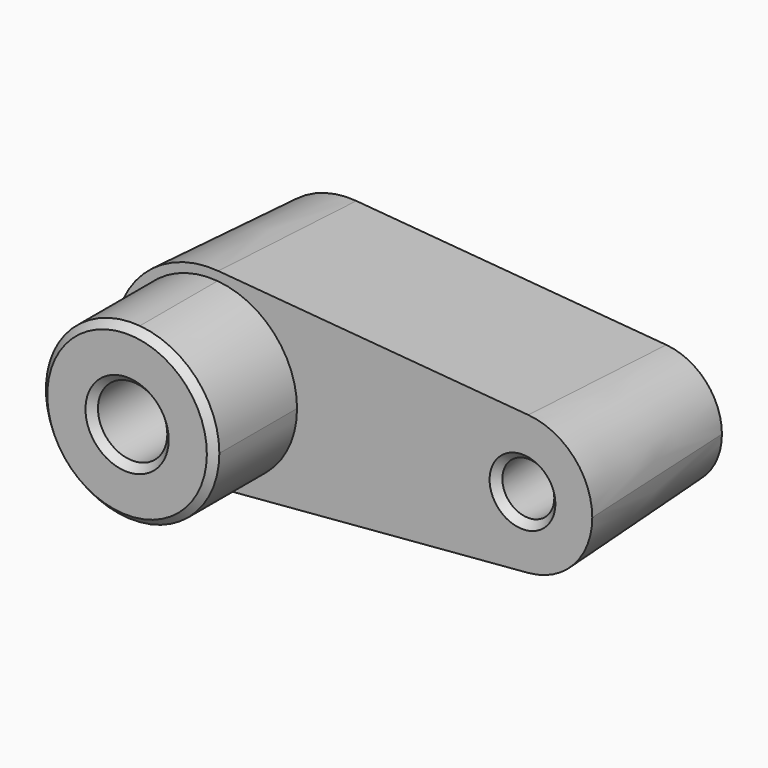
from build123d import *

# Parameters (mm, degrees)
F0_R     = 10
F1_DEPTH = 50
F1_TAPER = -3
F2_DEPTH = 80


# Not quite as in the source:
# - a fillet or chamfer that OpenCascade refuses, or shapes differently, is made with other operations: its cross-section is extruded or revolved along the edge and cut away or added


with BuildPart() as f1:
    # F0 (on Front) → F1 (new body)
    with BuildSketch(Plane.XZ):
        with BuildLine():
            ThreePointArc((2.0833333333, -24.9130432148), (18.3995018048, -16.9250800097), (25, 0))
            ThreePointArc((25, 0), (18.3995018048, 16.9250800097), (2.0833333333, 24.9130432148))
            ThreePointArc((2.0833333333, 24.9130432148), (-25, 0), (2.0833333333, -24.9130432148))
        make_face()
        Circle(F0_R, mode=Mode.SUBTRACT)
        with BuildLine():
            ThreePointArc((2.0833333333, 24.9130432148), (18.3995018048, 16.9250800097), (25, 0))
            ThreePointArc((25, 0), (18.3995018048, -16.9250800097), (2.0833333333, -24.9130432148))
            Line((2.0833333333, -24.9130432148), (91.4583333333, -17.4391302504))
            ThreePointArc((91.4583333333, -17.4391302504), (72.5, 0), (91.4583333333, 17.4391302504))
            Line((91.4583333333, 17.4391302504), (2.0833333333, 24.9130432148))
        make_face()
        with BuildLine():
            ThreePointArc((107.5, 0), (102.8796512634, 11.8475560068), (91.4583333333, 17.4391302504))
            ThreePointArc((91.4583333333, 17.4391302504), (72.5, 0), (91.4583333333, -17.4391302504))
            ThreePointArc((91.4583333333, -17.4391302504), (102.8796512634, -11.8475560068), (107.5, 0))
        make_face()
        with Locations((90, 0)):
            Circle(F0_R, mode=Mode.SUBTRACT)
    extrude(amount=F1_DEPTH, taper=F1_TAPER)

    # F0 (on Front) → F2 (join)
    with BuildSketch(Plane.XZ):
        with BuildLine():
            ThreePointArc((2.0833333333, -24.9130432148), (18.3995018048, -16.9250800097), (25, 0))
            ThreePointArc((25, 0), (18.3995018048, 16.9250800097), (2.0833333333, 24.9130432148))
            ThreePointArc((2.0833333333, 24.9130432148), (-25, 0), (2.0833333333, -24.9130432148))
        make_face()
        Circle(F0_R, mode=Mode.SUBTRACT)
    extrude(amount=F2_DEPTH)

    # F3: chamfer of 2 on 3 edges, made by hand

    # F3_s1 → F3_t2 (revolve, cut)
    with BuildSketch(Plane(origin=(0, 0, 0), x_dir=(0, 1, 0), z_dir=(0.9965217286, 0, 0.0833333333))):
        Polygon((-78, -25), (-80, -23), (-80, -25), align=None)
    revolve(axis=Axis((0, -80, 0), (0, 1, 0)), mode=Mode.SUBTRACT)

    # F3_s3 → F3_t4 (revolve, cut)
    with BuildSketch(Plane.XY):
        Polygon((12, -80), (10, -78), (10, -80), align=None)
    revolve(axis=Axis((0, -80, 0), (0, -1, 0)), mode=Mode.SUBTRACT)

    # F3_s5 → F3_t6 (revolve, cut)
    with BuildSketch(Plane.XY):
        Polygon((99.4871712864, -50), (97.4899122169, -47.8953280875), (97.3796110358, -50), align=None)
    revolve(axis=Axis((90, -50, 0), (0, 1, 0)), mode=Mode.SUBTRACT)


solid = f1.part
